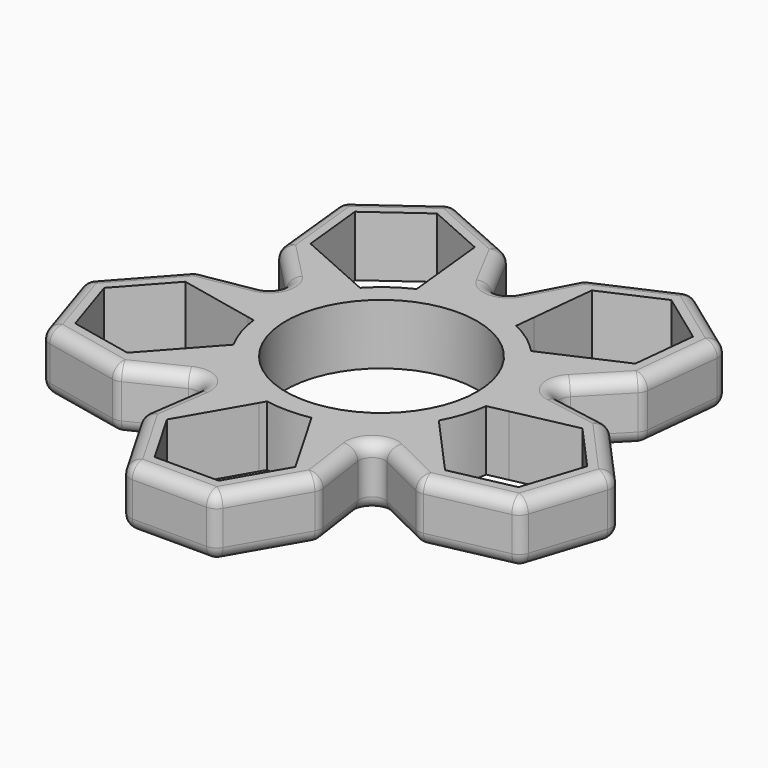
from build123d import *

# Parameters (mm, degrees)
F0_R     = 11.1
F1_DEPTH = 3.5
F2_DEPTH = 3.5
F3_R     = 1.5


with BuildPart() as f1:
    # F0 (on Top) → F1 (new body, symmetric)
    with BuildSketch(Plane.XY):
        with BuildLine():
            ThreePointArc((13.1839352073, 3.3382409216), (12.9334883923, 4.2053392261), (12.6260811493, 5.0539167793))
            ThreePointArc((12.6260811493, 5.0539167793), (11.475161525, 7.2993607923), (9.9292475091, 9.2935485098))
            ThreePointArc((9.9292475091, 9.2935485098), (7.9938794312, 11.0026311235), (5.7703836481, 12.315139973))
            ThreePointArc((5.7703836481, 12.315139973), (3.3933272935, 13.1698644594), (0.8992042504, 13.5702406654))
            ThreePointArc((0.8992042504, 13.5702406654), (-0.0028475645, 13.5999997019), (-0.9048868383, 13.5698629252))
            ThreePointArc((-0.9048868383, 13.5698629252), (-3.3960847219, 13.1691536767), (-5.7703836481, 12.315139973))
            ThreePointArc((-5.7703836481, 12.315139973), (-7.9938794312, 11.0026311235), (-9.9292475091, 9.2935485098))
            ThreePointArc((-9.9292475091, 9.2935485098), (-11.4766896117, 7.296957966), (-12.6281964177, 5.0486290451))
            ThreePointArc((-12.6281964177, 5.0486290451), (-12.9352482839, 4.1999228366), (-13.1853319713, 3.3327197311))
            ThreePointArc((-13.1853319713, 3.3327197311), (-13.5740573118, 0.839623783), (-13.4955407317, -1.6823734303))
            ThreePointArc((-13.4955407317, -1.6823734303), (-12.9343686216, -4.2026311235), (-11.9069960914, -6.5714111178))
            ThreePointArc((-11.9069960914, -6.5714111178), (-10.4863115518, -8.660096422), (-8.7038588531, -10.4500163189))
            Line((-8.7038588531, -10.4500163189), (-8.7033351883, -10.4463705793))
            add(Edge.make_bspline(
                [(-8.7033351883, -10.4463705793), (-2.9857461341, -11.7604713887), (3.0112343375, -11.9255259633), (8.7082341333, -10.4463705793)],
                knots=[0, 0, 0, 0, 17.4115693216, 17.4115693216, 17.4115693216, 17.4115693216], degree=3))
            ThreePointArc((8.7082341333, -10.4463705793), (10.4881245707, -8.6579006109), (11.9069960914, -6.5714111178))
            ThreePointArc((11.9069960914, -6.5714111178), (12.9343686216, -4.2026311235), (13.4955407317, -1.6823734303))
            ThreePointArc((13.4955407317, -1.6823734303), (13.5738600617, -0.8428066352), (13.6, 0))
            ThreePointArc((13.6, 0), (13.4955829592, 1.682034658), (13.1839352073, 3.3382409216))
        make_face()
        Circle(F0_R, mode=Mode.SUBTRACT)
        with BuildLine():
            ThreePointArc((7.2489158132, -11.5070943132), (7.996182984, -11.0009571259), (8.7082341333, -10.4463705793))
            add(Edge.make_bspline(
                [(-8.7033351883, -10.4463705793), (-2.9857461341, -11.7604713887), (3.0112343375, -11.9255259633), (8.7082341333, -10.4463705793)],
                knots=[0, 0, 0, 0, 17.4115693216, 17.4115693216, 17.4115693216, 17.4115693216], degree=3))
            Line((-8.7033351883, -10.4463705793), (-8.7038588531, -10.4500163189))
            ThreePointArc((-8.7038588531, -10.4500163189), (-7.9915755279, -11.0043046387), (-7.2440964729, -11.5101288564))
            ThreePointArc((-7.2440964729, -11.5101288564), (-4.993144062, -12.6502376411), (-2.5703192207, -13.3549039347))
            ThreePointArc((-2.5703192207, -13.3549039347), (0, -13.6), (2.5703192207, -13.3549039347))
            ThreePointArc((2.5703192207, -13.3549039347), (4.995792656, -12.6491919006), (7.2489158132, -11.5070943132))
        make_face()
    extrude(amount=F1_DEPTH, both=True)

    # F0 (on Top) → F2 (join, symmetric)
    with BuildSketch(Plane.XY):
        with BuildLine():
            Line((8.9821286946, -12.3589607707), (7.2489158132, -11.5070943132))
            ThreePointArc((7.2489158132, -11.5070943132), (4.995792656, -12.6491919006), (2.5703192207, -13.3549039347))
            Line((2.5703192207, -13.3549039347), (3.7239092363, -15.3529804528))
            Line((3.7239092363, -15.3529804528), (7.4478184725, -21.8029804528))
            Line((7.4478184725, -21.8029804528), (3.7239092363, -28.2529804528))
            Line((3.7239092363, -28.2529804528), (-3.7239092363, -28.2529804528))
            Line((-3.7239092363, -28.2529804528), (-7.4478184725, -21.8029804528))
            Line((-7.4478184725, -21.8029804528), (-2.9648464341, -14.0382451132))
            Line((-2.9648464341, -14.0382451132), (-2.5703192207, -13.3549039347))
            ThreePointArc((-2.5703192207, -13.3549039347), (-4.993144062, -12.6502376411), (-7.2440964729, -11.5101288564))
            Line((-7.2440964729, -11.5101288564), (-8.9784397633, -12.3616409361))
            Line((-8.9784397633, -12.3616409361), (-10.3345698185, -21.8029804528))
            Line((-10.3345698185, -21.8029804528), (-5.1672849092, -30.7529804528))
            Line((-5.1672849092, -30.7529804528), (5.1672849092, -30.7529804528))
            Line((5.1672849092, -30.7529804528), (10.3345698185, -21.8029804528))
            Line((10.3345698185, -21.8029804528), (8.9821286946, -12.3589607707))
        make_face()
        with BuildLine():
            ThreePointArc((7.2489158132, -11.5070943132), (7.996182984, -11.0009571259), (8.7082341333, -10.4463705793))
            add(Edge.make_bspline(
                [(-8.7033351883, -10.4463705793), (-2.9857461341, -11.7604713887), (3.0112343375, -11.9255259633), (8.7082341333, -10.4463705793)],
                knots=[0, 0, 0, 0, 17.4115693216, 17.4115693216, 17.4115693216, 17.4115693216], degree=3))
            Line((-8.7033351883, -10.4463705793), (-8.7038588531, -10.4500163189))
            ThreePointArc((-8.7038588531, -10.4500163189), (-7.9915755279, -11.0043046387), (-7.2440964729, -11.5101288564))
            ThreePointArc((-7.2440964729, -11.5101288564), (-4.993144062, -12.6502376411), (-2.5703192207, -13.3549039347))
            ThreePointArc((-2.5703192207, -13.3549039347), (0, -13.6), (2.5703192207, -13.3549039347))
            ThreePointArc((2.5703192207, -13.3549039347), (4.995792656, -12.6491919006), (7.2489158132, -11.5070943132))
        make_face()
        with BuildLine():
            ThreePointArc((-7.2440964729, -11.5101288564), (-7.9915755279, -11.0043046387), (-8.7038588531, -10.4500163189))
            Line((-8.7038588531, -10.4500163189), (-8.9784397633, -12.3616409361))
            Line((-8.9784397633, -12.3616409361), (-7.2440964729, -11.5101288564))
        make_face()
        with BuildLine():
            Line((-8.9784397633, -12.3616409361), (-8.7038588531, -10.4500163189))
            ThreePointArc((-8.7038588531, -10.4500163189), (-10.4863115518, -8.660096422), (-11.9069960914, -6.5714111178))
            Line((-11.9069960914, -6.5714111178), (-13.4508008646, -8.2859800195))
            Line((-13.4508008646, -8.2859800195), (-18.4343641552, -13.8207877784))
            Line((-18.4343641552, -13.8207877784), (-25.7194299249, -12.2722992469))
            Line((-25.7194299249, -12.2722992469), (-28.0209324039, -5.1890029564))
            Line((-28.0209324039, -5.1890029564), (-23.0373691133, 0.3458048026))
            Line((-23.0373691133, 0.3458048026), (-14.2673524261, -1.5183197903))
            Line((-14.2673524261, -1.5183197903), (-13.4955407317, -1.6823734303))
            ThreePointArc((-13.4955407317, -1.6823734303), (-13.5740573118, 0.839623783), (-13.1853319713, 3.3327197311))
            Line((-13.1853319713, 3.3327197311), (-14.5311096343, 4.7190465154))
            Line((-14.5311096343, 4.7190465154), (-23.9294243377, 3.0912684811))
            Line((-23.9294243377, 3.0912684811), (-30.8446013068, -4.5888136031))
            Line((-30.8446013068, -4.5888136031), (-27.6510436034, -14.4175735721))
            Line((-27.6510436034, -14.4175735721), (-17.5423089308, -16.5662514569))
            Line((-17.5423089308, -16.5662514569), (-8.9784397633, -12.3616409361))
        make_face()
        with BuildLine():
            ThreePointArc((-13.1853319713, 3.3327197311), (-12.9352482839, 4.1999228366), (-12.6281964177, 5.0486290451))
            Line((-12.6281964177, 5.0486290451), (-14.5311096343, 4.7190465154))
            Line((-14.5311096343, 4.7190465154), (-13.1853319713, 3.3327197311))
        make_face()
        with BuildLine():
            ThreePointArc((-5.7703836481, 12.315139973), (-3.3960847219, 13.1691536767), (-0.9048868383, 13.5698629252))
            Line((-0.9048868383, 13.5698629252), (-0.0022798849, 15.2781720772))
            Line((-0.0022798849, 15.2781720772), (-4.4546277534, 23.7134894424))
            Line((-4.4546277534, 23.7134894424), (-13.8957270678, 27.916937678))
            Line((-13.8957270678, 27.916937678), (-22.2565696805, 21.8424299499))
            Line((-22.2565696805, 21.8424299499), (-21.1763129789, 11.5644739862))
            Line((-21.1763129789, 11.5644739862), (-14.5311096343, 4.7190465154))
            Line((-14.5311096343, 4.7190465154), (-12.6281964177, 5.0486290451))
            ThreePointArc((-12.6281964177, 5.0486290451), (-11.4766896117, 7.296957966), (-9.9292475091, 9.2935485098))
            Line((-9.9292475091, 9.2935485098), (-12.0369613465, 10.2319631706))
            Line((-12.0369613465, 10.2319631706), (-18.8408820815, 13.2612638544))
            Line((-18.8408820815, 13.2612638544), (-19.6193911011, 20.6682823981))
            Line((-19.6193911011, 20.6682823981), (-13.5939793858, 25.046000258))
            Line((-13.5939793858, 25.046000258), (-6.7900586509, 22.0166995742))
            Line((-6.7900586509, 22.0166995742), (-5.8528622947, 13.099871877))
            Line((-5.8528622947, 13.099871877), (-5.7703836481, 12.315139973))
        make_face()
        with BuildLine():
            Line((14.5297005879, 4.7233831142), (12.6260811493, 5.0539167793))
            ThreePointArc((12.6260811493, 5.0539167793), (12.9334883923, 4.2053392261), (13.1839352073, 3.3382409216))
            Line((13.1839352073, 3.3382409216), (14.5297005879, 4.7233831142))
        make_face()
        with BuildLine():
            Line((14.5297005879, 4.7233831142), (13.1839352073, 3.3382409216))
            ThreePointArc((13.1839352073, 3.3382409216), (13.4955829592, 1.682034658), (13.6, 0))
            ThreePointArc((13.6, 0), (13.5738600617, -0.8428066352), (13.4955407317, -1.6823734303))
            Line((13.4955407317, -1.6823734303), (15.7523033437, -1.202683729))
            Line((15.7523033437, -1.202683729), (23.0373691133, 0.3458048026))
            Line((23.0373691133, 0.3458048026), (28.0209324039, -5.1890029564))
            Line((28.0209324039, -5.1890029564), (25.7194299249, -12.2722992469))
            Line((25.7194299249, -12.2722992469), (18.4343641552, -13.8207877784))
            Line((18.4343641552, -13.8207877784), (12.4349765584, -7.1577928321))
            Line((12.4349765584, -7.1577928321), (11.9069960914, -6.5714111178))
            ThreePointArc((11.9069960914, -6.5714111178), (10.4881245707, -8.6579006109), (8.7082341333, -10.4463705793))
            Line((8.7082341333, -10.4463705793), (8.9821286946, -12.3589607707))
            Line((8.9821286946, -12.3589607707), (17.5423089308, -16.5662514569))
            Line((17.5423089308, -16.5662514569), (27.6510436034, -14.4175735721))
            Line((27.6510436034, -14.4175735721), (30.8446013068, -4.5888136031))
            Line((30.8446013068, -4.5888136031), (23.9294243377, 3.0912684811))
            Line((23.9294243377, 3.0912684811), (14.5297005879, 4.7233831142))
        make_face()
        with BuildLine():
            Line((8.9821286946, -12.3589607707), (8.7082341333, -10.4463705793))
            ThreePointArc((8.7082341333, -10.4463705793), (7.996182984, -11.0009571259), (7.2489158132, -11.5070943132))
            Line((7.2489158132, -11.5070943132), (8.9821286946, -12.3589607707))
        make_face()
        with BuildLine():
            ThreePointArc((9.9292475091, 9.2935485098), (11.475161525, 7.2993607923), (12.6260811493, 5.0539167793))
            Line((12.6260811493, 5.0539167793), (14.5297005879, 4.7233831142))
            Line((14.5297005879, 4.7233831142), (21.1763129789, 11.5644739862))
            Line((21.1763129789, 11.5644739862), (22.2565696805, 21.8424299499))
            Line((22.2565696805, 21.8424299499), (13.8957270678, 27.916937678))
            Line((13.8957270678, 27.916937678), (4.4546277534, 23.7134894424))
            Line((4.4546277534, 23.7134894424), (-0.0022798849, 15.2781720772))
            Line((-0.0022798849, 15.2781720772), (0.8992042504, 13.5702406654))
            ThreePointArc((0.8992042504, 13.5702406654), (3.3933272935, 13.1698644594), (5.7703836481, 12.315139973))
            Line((5.7703836481, 12.315139973), (6.0115496312, 14.6096810306))
            Line((6.0115496312, 14.6096810306), (6.7900586509, 22.0166995742))
            Line((6.7900586509, 22.0166995742), (13.5939793858, 25.046000258))
            Line((13.5939793858, 25.046000258), (19.6193911011, 20.6682823981))
            Line((19.6193911011, 20.6682823981), (18.8408820815, 13.2612638544))
            Line((18.8408820815, 13.2612638544), (10.6500845965, 9.6144858585))
            Line((10.6500845965, 9.6144858585), (9.9292475091, 9.2935485098))
        make_face()
        with BuildLine():
            ThreePointArc((-0.9048868383, 13.5698629252), (-0.0028475645, 13.5999997019), (0.8992042504, 13.5702406654))
            Line((0.8992042504, 13.5702406654), (-0.0022798849, 15.2781720772))
            Line((-0.0022798849, 15.2781720772), (-0.9048868383, 13.5698629252))
        make_face()
    extrude(amount=F2_DEPTH, both=True)

    # F3
    f3_edges = [f1.edges().sort_by_distance(p)[0] for p in [
        (-22.25657, 21.84243, 0),
        (-21.716441, 16.703452, -3.5),
        (-21.176313, 11.564474, 0),
        (-21.716441, 16.703452, 3.5),
        (-17.853711, 8.14176, -3.5),
        (-14.53111, 4.719047, 0),
        (-17.853711, 8.14176, 3.5),
        (-13.895727, 27.916938, 0),
        (-18.076148, 24.879684, -3.5),
        (-18.076148, 24.879684, 3.5),
        (-23.929424, 3.091268, 0),
        (-27.387013, -0.748773, -3.5),
        (-30.844601, -4.588814, 0),
        (-27.387013, -0.748773, 3.5),
        (-19.230267, 3.905157, -3.5),
        (-19.230267, 3.905157, 3.5),
        (-29.247822, -9.503194, -3.5),
        (-27.651044, -14.417574, 0),
        (-29.247822, -9.503194, 3.5),
        (-17.542309, -16.566251, 0),
        (-13.260374, -14.463946, -3.5),
        (-8.97844, -12.361641, 0),
        (-13.260374, -14.463946, 3.5),
        (-9.656505, -17.082311, -3.5),
        (-10.33457, -21.80298, 0),
        (-9.656505, -17.082311, 3.5),
        (-22.596676, -15.491913, -3.5),
        (-22.596676, -15.491913, 3.5),
        (-7.750927, -26.27798, -3.5),
        (-5.167285, -30.75298, 0),
        (-7.750927, -26.27798, 3.5),
        (0, -30.75298, -3.5),
        (5.167285, -30.75298, 0),
        (0, -30.75298, 3.5),
        (7.750927, -26.27798, -3.5),
        (10.33457, -21.80298, 0),
        (7.750927, -26.27798, 3.5),
        (9.658349, -17.080971, -3.5),
        (8.982129, -12.358961, 0),
        (9.658349, -17.080971, 3.5),
        (13.262219, -14.462606, -3.5),
        (17.542309, -16.566251, 0),
        (13.262219, -14.462606, 3.5),
        (22.596676, -15.491913, -3.5),
        (27.651044, -14.417574, 0),
        (22.596676, -15.491913, 3.5),
        (29.247822, -9.503194, -3.5),
        (30.844601, -4.588814, 0),
        (29.247822, -9.503194, 3.5),
        (27.387013, -0.748773, -3.5),
        (23.929424, 3.091268, 0),
        (27.387013, -0.748773, 3.5),
        (19.229562, 3.907326, -3.5),
        (14.529701, 4.723383, 0),
        (19.229562, 3.907326, 3.5),
        (17.853007, 8.143929, -3.5),
        (21.176313, 11.564474, 0),
        (17.853007, 8.143929, 3.5),
        (21.716441, 16.703452, -3.5),
        (22.25657, 21.84243, 0),
        (21.716441, 16.703452, 3.5),
        (18.076148, 24.879684, -3.5),
        (13.895727, 27.916938, 0),
        (18.076148, 24.879684, 3.5),
        (9.175177, 25.815214, -3.5),
        (4.454628, 23.713489, 0),
        (9.175177, 25.815214, 3.5),
        (2.226174, 19.495831, -3.5),
        (-0.00228, 15.278172, 0),
        (2.226174, 19.495831, 3.5),
        (-2.228454, 19.495831, -3.5),
        (-4.454628, 23.713489, 0),
        (-2.228454, 19.495831, 3.5),
        (-9.175177, 25.815214, -3.5),
        (-9.175177, 25.815214, 3.5),
    ]]
    fillet(f3_edges, radius=F3_R)


solid = f1.part
